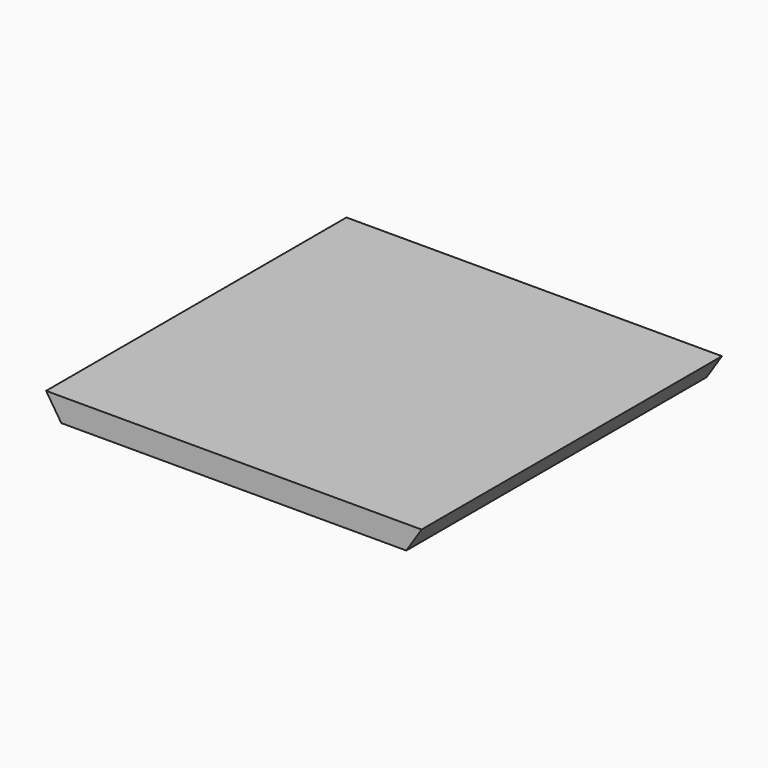
from build123d import *

# Parameters (mm, degrees)
F0_W       = 304.8
F0_H       = 304.8
F1_DEPTH   = 19.05
F2_SIZE2   = 12.371205
F2_SIZE    = 19.04999
F2_2_SIZE2 = 12.371205
F2_2_SIZE  = 19.04999


# Not quite as in the source:
# - a fillet or chamfer is up to 0.001 mm smaller than in the source, because OpenCascade refuses the exact size


with BuildPart() as f1:
    # F0 (on Top) → F1 (new body)
    with BuildSketch(Plane.XY):
        with Locations((3.4177321941, -5.1832514624)):
            Rectangle(F0_W, F0_H)
    extrude(amount=F1_DEPTH)

    # F2 (size 19.05 and 12.3712146504 in the source; OpenCascade refuses exactly that, so slightly less here)
    f2_edges = [f1.edges().sort_by_distance(p)[0] for p in [
        (-148.982268, -5.183251, 0),
    ]]
    f2_side = f1.faces().sort_by_distance((-148.982268, -5.183251, 9.525))[0]
    chamfer(f2_edges, length=F2_SIZE, length2=F2_SIZE2, reference=f2_side)

    # F2#2 (size 19.05 and 12.3712146504 in the source; OpenCascade refuses exactly that, so slightly less here)
    f2_2_edges = [f1.edges().sort_by_distance(p)[0] for p in [
        (155.817732, -5.183251, 0),
    ]]
    f2_2_side = f1.faces().sort_by_distance((155.817732, -5.183251, 9.525))[0]
    chamfer(f2_2_edges, length=F2_2_SIZE, length2=F2_2_SIZE2, reference=f2_2_side)


solid = f1.part
